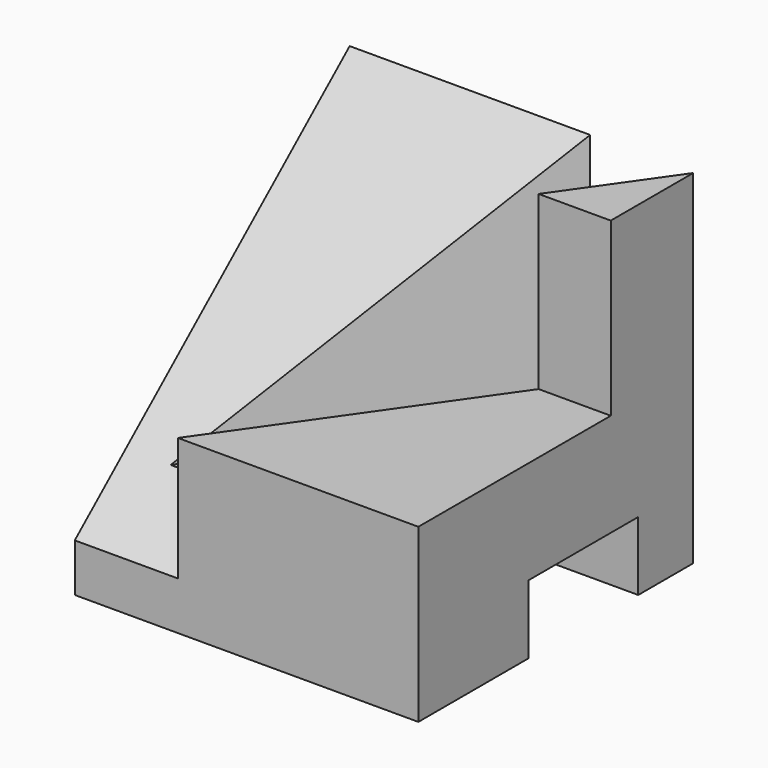
from build123d import *

# Parameters (mm, degrees)
F0_W      = 50
F0_H      = 50
F1_DEPTH  = 50
F3_DEPTH  = 43
F5_DEPTH  = 25
F6_DEPTH  = 43
F8_REACH  = 115.9479483752
F12_DEPTH = 35
F13_W     = 20
F13_H     = 10
F14_DEPTH = 30


with BuildPart() as f1:
    # F0 (on Front) → F1 (new body)
    with BuildSketch(Plane.XZ):
        with Locations((25, 25)):
            Rectangle(F0_W, F0_H)
    extrude(amount=F1_DEPTH)

    # F2 (on face) → F3 (cut)
    with BuildSketch(Plane.XY.offset(50)):
        Polygon((15, -50), (50, 0), (35, 0), (0, -50), align=None)
    extrude(amount=-F3_DEPTH, mode=Mode.SUBTRACT)

    # F4 (on face) → F5 (cut)
    with BuildSketch(Plane.XY.offset(50)):
        Polygon((50, -50), (50, -15), (39.5, -15), (15, -50), align=None)
    extrude(amount=-F5_DEPTH, mode=Mode.SUBTRACT)

    # F6 (cut): a face of the model
    f6_faces = [f1.faces().sort_by_distance(p)[0] for p in [
        (11.6666666667, -16.6666666667, 50),
    ]]
    extrude(f6_faces, amount=-F6_DEPTH, mode=Mode.SUBTRACT)

    f8_end = Plane(origin=(36.1029411765, -19.8529411765, 22.3235294118), x_dir=(-0.5734623444, -0.8192319205, 0), z_dir=(-0.8192319205, 0.5734623444, 0))
    # F7 (on face) → F8 (join, up to a plane its end follows)
    with BuildSketch(Plane(origin=(0, 0, 0), x_dir=(0, -1, 0), z_dir=(-1, 0, 0))):
        Polygon((50, 7), (0, 50), (0, 7), align=None)
    f8_long = extrude(amount=-F8_REACH, mode=Mode.PRIVATE)
    add(split(f8_long, bisect_by=f8_end, keep=Keep.TOP, mode=Mode.PRIVATE))

    # F10 (on plane+point) → F12 (cut, through all)
    with BuildSketch(Plane.XY.offset(50)):
        Polygon((15, -50), (50.0000000002, 0), (35.0000000002, 0), (0, -50), align=None)
    extrude(amount=-F12_DEPTH, mode=Mode.SUBTRACT)

    # F13 (on face) → F14 (cut)
    with BuildSketch(Plane.YZ.offset(50)):
        with Locations((-20, 5)):
            Rectangle(F13_W, F13_H)
    extrude(amount=-F14_DEPTH, mode=Mode.SUBTRACT)


solid = f1.part
